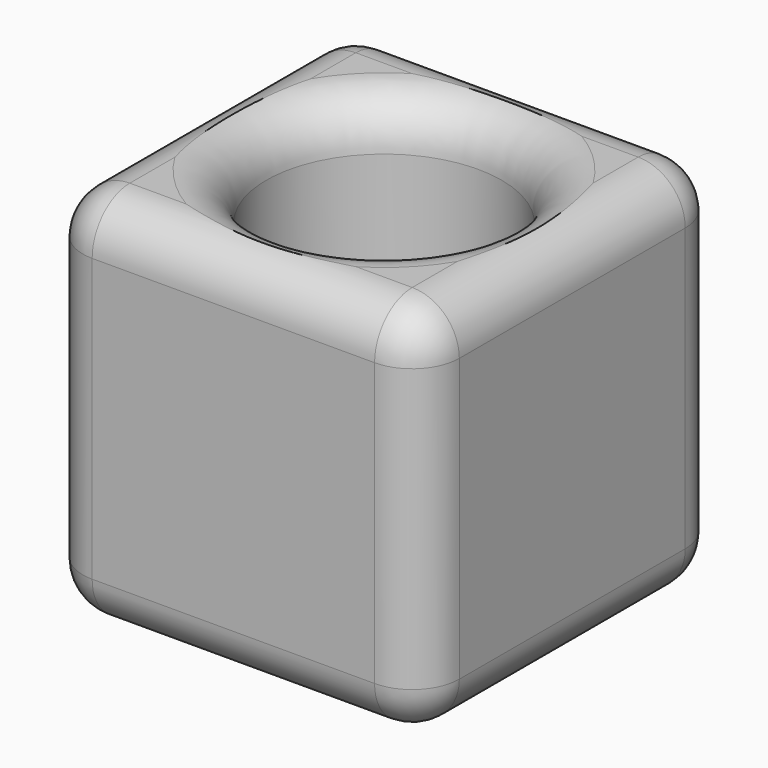
from build123d import *

# Parameters (mm, degrees)
F0_W          = 40
F0_H          = 40
F0_R          = 12.5
F1_DEPTH      = 20
F1_DEPTH_BACK = 20
F2_T1_DEPTH   = 30
F2_T3_DEPTH   = 30
F2_T5_DEPTH   = 30
F2_S9_W       = 5
F2_S9_H       = 5
F2_T10_DEPTH  = 5
F2_S15_W      = 5
F2_S15_H      = 5
F2_T16_DEPTH  = 5
F2_S21_W      = 5
F2_S21_H      = 5
F2_T22_DEPTH  = 5
F2_S27_W      = 5
F2_S27_H      = 5
F2_T28_DEPTH  = 5
F2_S33_W      = 5
F2_S33_H      = 5
F2_T34_DEPTH  = 5
F2_S39_W      = 5
F2_S39_H      = 5
F2_T40_DEPTH  = 5
F2_S45_W      = 5
F2_S45_H      = 5
F2_T46_DEPTH  = 5
F2_S51_W      = 5
F2_S51_H      = 5
F2_T52_DEPTH  = 5


# Not quite as in the source:
# - a fillet or chamfer that OpenCascade refuses, or shapes differently, is made with other operations: its cross-section is extruded or revolved along the edge and cut away or added


with BuildPart() as f1:
    # F0 (on Top) → F1 (new body, two sides)
    with BuildSketch(Plane.XY) as f1_sk:
        Rectangle(F0_W, F0_H)
        Circle(F0_R, mode=Mode.SUBTRACT)
    extrude(amount=F1_DEPTH)
    extrude(f1_sk.sketch, amount=-F1_DEPTH_BACK)

    # F2: fillet of radius 5 on 14 edges, made by hand

    # F2_s2 → F2_t1 (cut)
    with BuildSketch(Plane.XZ.offset(-15)):
        with BuildLine():
            ThreePointArc((20, 15), (18.5355339059, 18.5355339059), (15, 20))
            Line((15, 20), (20, 20))
            Line((20, 20), (20, 15))
        make_face()
        with BuildLine():
            ThreePointArc((-20, 15), (-18.5355339059, 18.5355339059), (-15, 20))
            Line((-15, 20), (-20, 20))
            Line((-20, 20), (-20, 15))
        make_face()
        with BuildLine():
            ThreePointArc((20, -15), (18.5355339059, -18.5355339059), (15, -20))
            Line((15, -20), (20, -20))
            Line((20, -20), (20, -15))
        make_face()
        with BuildLine():
            ThreePointArc((-15, -20), (-18.5355339059, -18.5355339059), (-20, -15))
            Line((-20, -15), (-20, -20))
            Line((-20, -20), (-15, -20))
        make_face()
    extrude(amount=F2_T1_DEPTH, mode=Mode.SUBTRACT)

    # F2_s4 → F2_t3 (cut)
    with BuildSketch(Plane.YZ.offset(-15)):
        with BuildLine():
            ThreePointArc((20, 15), (18.5355339059, 18.5355339059), (15, 20))
            Line((15, 20), (20, 20))
            Line((20, 20), (20, 15))
        make_face()
        with BuildLine():
            ThreePointArc((-15, 20), (-18.5355339059, 18.5355339059), (-20, 15))
            Line((-20, 15), (-20, 20))
            Line((-20, 20), (-15, 20))
        make_face()
        with BuildLine():
            ThreePointArc((15, -20), (18.5355339059, -18.5355339059), (20, -15))
            Line((20, -15), (20, -20))
            Line((20, -20), (15, -20))
        make_face()
        with BuildLine():
            ThreePointArc((-15, -20), (-18.5355339059, -18.5355339059), (-20, -15))
            Line((-20, -15), (-20, -20))
            Line((-20, -20), (-15, -20))
        make_face()
    extrude(amount=F2_T3_DEPTH, mode=Mode.SUBTRACT)

    # F2_s6 → F2_t5 (cut)
    with BuildSketch(Plane.XY.offset(-15)):
        with BuildLine():
            ThreePointArc((-20, 15), (-18.5355339059, 18.5355339059), (-15, 20))
            Line((-15, 20), (-20, 20))
            Line((-20, 20), (-20, 15))
        make_face()
        with BuildLine():
            ThreePointArc((20, 15), (18.5355339059, 18.5355339059), (15, 20))
            Line((15, 20), (20, 20))
            Line((20, 20), (20, 15))
        make_face()
        with BuildLine():
            ThreePointArc((-20, -15), (-18.5355339059, -18.5355339059), (-15, -20))
            Line((-15, -20), (-20, -20))
            Line((-20, -20), (-20, -15))
        make_face()
        with BuildLine():
            ThreePointArc((20, -15), (18.5355339059, -18.5355339059), (15, -20))
            Line((15, -20), (20, -20))
            Line((20, -20), (20, -15))
        make_face()
    extrude(amount=F2_T5_DEPTH, mode=Mode.SUBTRACT)


with BuildPart() as f2_tool8:
    # F2_s9 → F2_t10 (new body)
    with BuildSketch(Plane.YZ.offset(15)):
        with Locations((-17.5, 17.5)):
            Rectangle(F2_S9_W, F2_S9_H)
    extrude(amount=F2_T10_DEPTH)

    # F2_s11 → F2_t12 (revolve, cut)
    with BuildSketch(Plane(origin=(15, -15, 15), x_dir=(0, 0.7071067812, -0.7071067812), z_dir=(0, -0.7071067812, -0.7071067812))):
        with BuildLine():
            ThreePointArc((0, -5), (5, 0), (0, 5))
            Line((0, 5), (0, -5))
        make_face()
    revolve(axis=Axis((15, -15, 15), (1, 0, 0)), mode=Mode.SUBTRACT)


with BuildPart() as f1_1:
    add(f1.part)

    # F2_t7: cut F2_tool8
    add(f2_tool8.part, mode=Mode.SUBTRACT)


with BuildPart() as f2_tool14:
    # F2_s15 → F2_t16 (new body)
    with BuildSketch(Plane.YZ.offset(15)):
        with Locations((17.5, 17.5)):
            Rectangle(F2_S15_W, F2_S15_H)
    extrude(amount=F2_T16_DEPTH)

    # F2_s17 → F2_t18 (revolve, cut)
    with BuildSketch(Plane(origin=(15, 15, 15), x_dir=(0, -0.7071067812, -0.7071067812), z_dir=(0, -0.7071067812, 0.7071067812))):
        with BuildLine():
            ThreePointArc((0, -5), (5, 0), (0, 5))
            Line((0, 5), (0, -5))
        make_face()
    revolve(axis=Axis((15, 15, 15), (1, 0, 0)), mode=Mode.SUBTRACT)


with BuildPart() as f1_2:
    add(f1_1.part)

    # F2_t13: cut F2_tool14
    add(f2_tool14.part, mode=Mode.SUBTRACT)


with BuildPart() as f2_tool20:
    # F2_s21 → F2_t22 (new body)
    with BuildSketch(Plane.YZ.offset(-15)):
        with Locations((17.5, 17.5)):
            Rectangle(F2_S21_W, F2_S21_H)
    extrude(amount=-F2_T22_DEPTH)

    # F2_s23 → F2_t24 (revolve, cut)
    with BuildSketch(Plane(origin=(-15, 15, 15), x_dir=(0, -0.7071067812, -0.7071067812), z_dir=(0, 0.7071067812, -0.7071067812))):
        with BuildLine():
            ThreePointArc((0, -5), (5, 0), (0, 5))
            Line((0, 5), (0, -5))
        make_face()
    revolve(axis=Axis((-15, 15, 15), (-1, 0, 0)), mode=Mode.SUBTRACT)


with BuildPart() as f1_3:
    add(f1_2.part)

    # F2_t19: cut F2_tool20
    add(f2_tool20.part, mode=Mode.SUBTRACT)


with BuildPart() as f2_tool26:
    # F2_s27 → F2_t28 (new body)
    with BuildSketch(Plane.YZ.offset(-15)):
        with Locations((-17.5, 17.5)):
            Rectangle(F2_S27_W, F2_S27_H)
    extrude(amount=-F2_T28_DEPTH)

    # F2_s29 → F2_t30 (revolve, cut)
    with BuildSketch(Plane(origin=(-15, -15, 15), x_dir=(0, 0.7071067812, -0.7071067812), z_dir=(0, 0.7071067812, 0.7071067812))):
        with BuildLine():
            ThreePointArc((0, -5), (5, 0), (0, 5))
            Line((0, 5), (0, -5))
        make_face()
    revolve(axis=Axis((-15, -15, 15), (-1, 0, 0)), mode=Mode.SUBTRACT)


with BuildPart() as f1_4:
    add(f1_3.part)

    # F2_t25: cut F2_tool26
    add(f2_tool26.part, mode=Mode.SUBTRACT)


with BuildPart() as f2_tool32:
    # F2_s33 → F2_t34 (new body)
    with BuildSketch(Plane.XY.offset(-15)):
        with Locations((-17.5, 17.5)):
            Rectangle(F2_S33_W, F2_S33_H)
    extrude(amount=-F2_T34_DEPTH)

    # F2_s35 → F2_t36 (revolve, cut)
    with BuildSketch(Plane(origin=(-15, 15, -15), x_dir=(0.7071067812, -0.7071067812, 0), z_dir=(0.7071067812, 0.7071067812, 0))):
        with BuildLine():
            ThreePointArc((0, -5), (5, 0), (0, 5))
            Line((0, 5), (0, -5))
        make_face()
    revolve(axis=Axis((-15, 15, -15), (0, 0, -1)), mode=Mode.SUBTRACT)


with BuildPart() as f1_5:
    add(f1_4.part)

    # F2_t31: cut F2_tool32
    add(f2_tool32.part, mode=Mode.SUBTRACT)


with BuildPart() as f2_tool38:
    # F2_s39 → F2_t40 (new body)
    with BuildSketch(Plane.YZ.offset(15)):
        with Locations((17.5, -17.5)):
            Rectangle(F2_S39_W, F2_S39_H)
    extrude(amount=F2_T40_DEPTH)

    # F2_s41 → F2_t42 (revolve, cut)
    with BuildSketch(Plane(origin=(15, 15, -15), x_dir=(0, -0.7071067812, 0.7071067812), z_dir=(0, 0.7071067812, 0.7071067812))):
        with BuildLine():
            ThreePointArc((0, -5), (5, 0), (0, 5))
            Line((0, 5), (0, -5))
        make_face()
    revolve(axis=Axis((15, 15, -15), (1, 0, 0)), mode=Mode.SUBTRACT)


with BuildPart() as f1_6:
    add(f1_5.part)

    # F2_t37: cut F2_tool38
    add(f2_tool38.part, mode=Mode.SUBTRACT)


with BuildPart() as f2_tool44:
    # F2_s45 → F2_t46 (new body)
    with BuildSketch(Plane.YZ.offset(15)):
        with Locations((-17.5, -17.5)):
            Rectangle(F2_S45_W, F2_S45_H)
    extrude(amount=F2_T46_DEPTH)

    # F2_s47 → F2_t48 (revolve, cut)
    with BuildSketch(Plane(origin=(15, -15, -15), x_dir=(0, 0.7071067812, 0.7071067812), z_dir=(0, 0.7071067812, -0.7071067812))):
        with BuildLine():
            ThreePointArc((0, -5), (5, 0), (0, 5))
            Line((0, 5), (0, -5))
        make_face()
    revolve(axis=Axis((15, -15, -15), (1, 0, 0)), mode=Mode.SUBTRACT)


with BuildPart() as f1_7:
    add(f1_6.part)

    # F2_t43: cut F2_tool44
    add(f2_tool44.part, mode=Mode.SUBTRACT)


with BuildPart() as f2_tool50:
    # F2_s51 → F2_t52 (new body)
    with BuildSketch(Plane.XY.offset(-15)):
        with Locations((-17.5, -17.5)):
            Rectangle(F2_S51_W, F2_S51_H)
    extrude(amount=-F2_T52_DEPTH)

    # F2_s53 → F2_t54 (revolve, cut)
    with BuildSketch(Plane(origin=(-15, -15, -15), x_dir=(0.7071067812, 0.7071067812, 0), z_dir=(-0.7071067812, 0.7071067812, 0))):
        with BuildLine():
            ThreePointArc((0, -5), (5, 0), (0, 5))
            Line((0, 5), (0, -5))
        make_face()
    revolve(axis=Axis((-15, -15, -15), (0, 0, -1)), mode=Mode.SUBTRACT)


with BuildPart() as f1_8:
    add(f1_7.part)

    # F2_t49: cut F2_tool50
    add(f2_tool50.part, mode=Mode.SUBTRACT)

    # F2_s55 → F2_t56 (revolve, cut)
    with BuildSketch(Plane.XZ):
        with BuildLine():
            ThreePointArc((12.5, 15), (13.9644660941, 18.5355339059), (17.5, 20))
            Line((17.5, 20), (12.5, 20))
            Line((12.5, 20), (12.5, 15))
        make_face()
    revolve(axis=Axis((0, 0, 20), (0, 0, 1)), mode=Mode.SUBTRACT)

    # F2_s57 → F2_t58 (revolve, cut)
    with BuildSketch(Plane.XZ):
        with BuildLine():
            ThreePointArc((17.5, -20), (13.9644660941, -18.5355339059), (12.5, -15))
            Line((12.5, -15), (12.5, -20))
            Line((12.5, -20), (17.5, -20))
        make_face()
    revolve(axis=Axis((0, 0, -20), (0, 0, 1)), mode=Mode.SUBTRACT)


solid = f1_8.part
